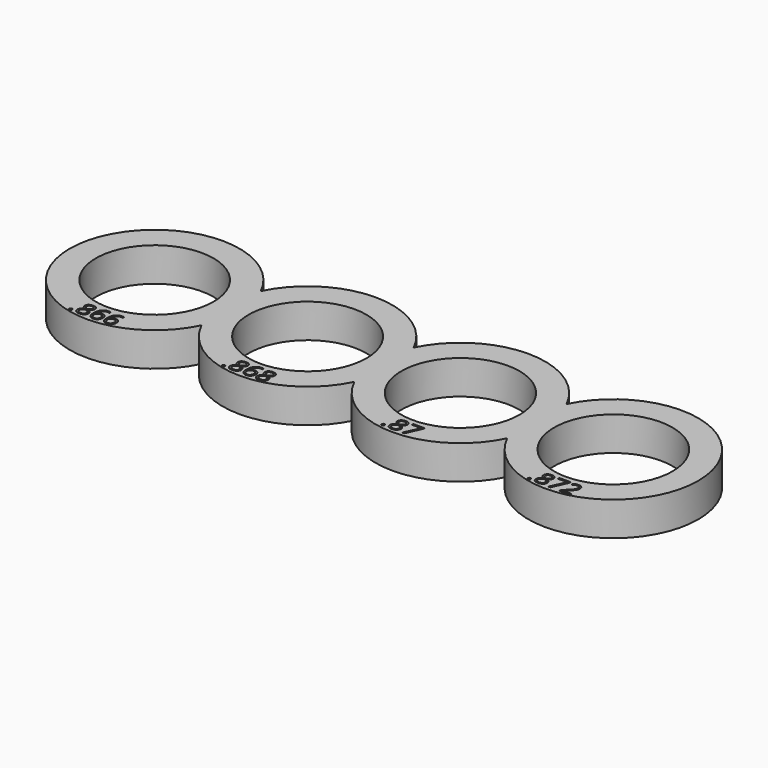
from build123d import *

# Parameters (mm, degrees)
F0_R         = 10.9982
F0_R_2       = 11.0236
F0_R_3       = 11.049
F0_R_4       = 11.0744
F1_DEPTH     = 6.35
F2_TEXT_SIZE = 4.4097222222
F3_DEPTH     = 1.5875


# Not quite as in the source:
# - Text() gives the source's letters only with a copy of the font that has no kerning and outlines rounded to 1/6400 em; it was checked with that copy


with BuildPart() as f1:
    # F0 (on Top) → F1 (new body)
    with BuildSketch(Plane.XY):
        with BuildLine():
            ThreePointArc((42.8625, 6.9197520729), (28.575, 15.875), (14.2875, 6.9197520729))
            ThreePointArc((14.2875, 6.9197520729), (-15.875, 0), (14.2875, -6.9197520729))
            ThreePointArc((14.2875, -6.9197520729), (28.575, -15.875), (42.8625, -6.9197520729))
            ThreePointArc((42.8625, -6.9197520729), (57.15, -15.875), (71.4375, -6.9197520729))
            ThreePointArc((71.4375, -6.9197520729), (101.6, 0), (71.4375, 6.9197520729))
            ThreePointArc((71.4375, 6.9197520729), (57.15, 15.875), (42.8625, 6.9197520729))
        make_face()
        Circle(F0_R, mode=Mode.SUBTRACT)
        with Locations((28.575, 0)):
            Circle(F0_R_2, mode=Mode.SUBTRACT)
        with Locations((57.15, 0)):
            Circle(F0_R_3, mode=Mode.SUBTRACT)
        with Locations((85.725, 0)):
            Circle(F0_R_4, mode=Mode.SUBTRACT)
    extrude(amount=F1_DEPTH)

    # F2 (on face) → F3 (cut)
    with BuildSketch(Plane.XY.offset(6.35)):
        with Locations((-4.4038655599, -15.113)):
            Text('.866', F2_TEXT_SIZE, font='Open Sans', text_align=(TextAlign.LEFT, TextAlign.BOTTOM))
        with Locations((24.1776801215, -15.113)):
            Text('.868', F2_TEXT_SIZE, font='Open Sans', text_align=(TextAlign.LEFT, TextAlign.BOTTOM))
        with Locations((54.0111735026, -15.113)):
            Text('.87', F2_TEXT_SIZE, font='Open Sans', text_align=(TextAlign.LEFT, TextAlign.BOTTOM))
        with Locations((81.3318142361, -15.113)):
            Text('.872', F2_TEXT_SIZE, font='Open Sans', text_align=(TextAlign.LEFT, TextAlign.BOTTOM))
    extrude(amount=-F3_DEPTH, mode=Mode.SUBTRACT)


solid = f1.part
